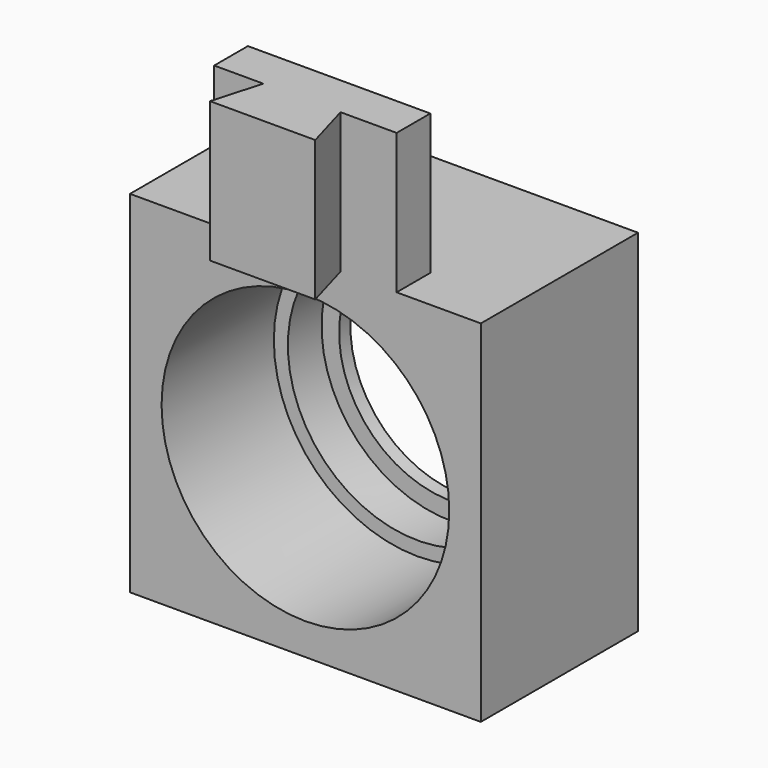
from build123d import *

# Parameters (mm, degrees)
F0_W      = 25
F0_H      = 25
F0_R      = 10.25
F0_R_2    = 9.25
F0_R_3    = 8
F1_DEPTH  = 1
F2_W      = 25
F2_H      = 25
F2_R      = 9.25
F3_DEPTH  = 3
F4_W      = 25
F4_H      = 25
F4_R      = 10.25
F5_DEPTH  = 10
F6_W      = 13
F6_H      = 3
F7_DEPTH  = 10
F8_W      = 7.5
F8_H      = 10
F9_DEPTH  = 3.5
F11_DEPTH = 10
F12_DEPTH = 10


with BuildPart() as f1:
    # F0 (on Front) → F1 (new body)
    with BuildSketch(Plane.XZ):
        with Locations((12.5, 12.5)):
            Rectangle(F0_W, F0_H)
        with Locations((12.5, 12.5)):
            Circle(F0_R, mode=Mode.SUBTRACT)
        with Locations((12.5, 12.5)):
            Circle(F0_R)
        with Locations((12.5, 12.5)):
            Circle(F0_R_2, mode=Mode.SUBTRACT)
        with Locations((12.5, 12.5)):
            Circle(F0_R_2)
        with Locations((12.5, 12.5)):
            Circle(F0_R_3, mode=Mode.SUBTRACT)
    extrude(amount=F1_DEPTH)

    # F2 (on face) → F3 (join)
    with BuildSketch(Plane.XZ.offset(1)):
        with Locations((12.5, 12.5)):
            Rectangle(F2_W, F2_H)
        with Locations((12.5, 12.5)):
            Circle(F2_R, mode=Mode.SUBTRACT)
    extrude(amount=F3_DEPTH)

    # F4 (on face) → F5 (join)
    with BuildSketch(Plane.XZ.offset(4)):
        with Locations((12.5, 12.5)):
            Rectangle(F4_W, F4_H)
        with Locations((12.5, 12.5)):
            Circle(F4_R, mode=Mode.SUBTRACT)
    extrude(amount=F5_DEPTH)

    # F6 (on face) → F7 (join)
    with BuildSketch(Plane.XY.offset(25)):
        with Locations((12.5, -12.5)):
            Rectangle(F6_W, F6_H)
    extrude(amount=F7_DEPTH)

    # F8 (on face) → F9 (join)
    with BuildSketch(Plane.XZ.offset(14)):
        with Locations((12.25, 30)):
            Rectangle(F8_W, F8_H)
    extrude(amount=F9_DEPTH)

    # F10 (on face) → F11 (cut)
    with BuildSketch(Plane.XY.offset(35)):
        Polygon((8.5, -14), (8.5, -17.5), (9.5, -14), align=None)
    extrude(amount=-F11_DEPTH, mode=Mode.SUBTRACT)

    # F10 (on face) → F12 (cut)
    with BuildSketch(Plane.XY.offset(35)):
        Polygon((15, -14), (16, -17.5), (16, -14), align=None)
    extrude(amount=-F12_DEPTH, mode=Mode.SUBTRACT)


solid = f1.part
